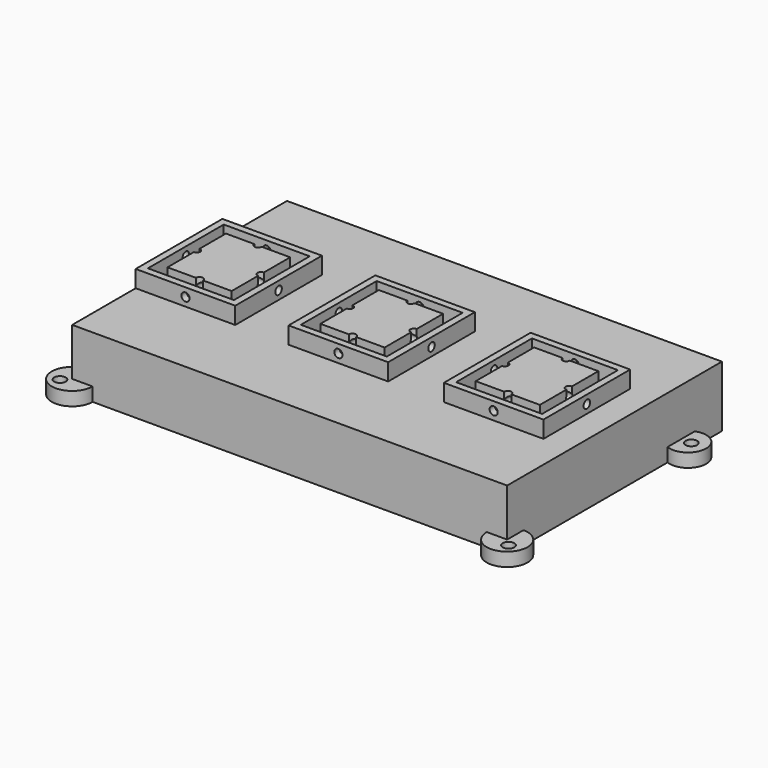
from build123d import *

# Parameters (mm, degrees)
F0_W         = 124
F0_H         = 75
F0_R         = 2
F1_DEPTH     = 2
F2_DEPTH     = 18
F3_W         = 124
F3_H         = 14
F4_DEPTH     = 2
F5_DEPTH     = 5
F6_W         = 124
F6_H         = 1
F7_DEPTH     = 75
F8_W         = 29.3
F8_H         = 31.9
F8_W_2       = 25.3
F8_H_2       = 27.9
F9_DEPTH     = 5
F10_DEPTH    = 4
F11_D        = 3.4
F13_D        = 2.4
F17_D        = 2.4
F17_ON_F15_D = 2.4
F17_ON_F16_D = 2.4
F18_R        = 1.5
F19_DEPTH    = 2


# Not quite as in the source:
# - a feature names something its author has since deleted; it is built from what else it names


with BuildPart() as f1:
    # F0 (on Top) → F1 (new body)
    with BuildSketch(Plane.XY):
        with Locations((1.9529018402, -1.4505029619)):
            Rectangle(F0_W, F0_H)
        with Locations((-53.0470981598, -18.9505029619)):
            Circle(F0_R, mode=Mode.SUBTRACT)
        with Locations((56.9529018402, -18.9505029619)):
            Circle(F0_R, mode=Mode.SUBTRACT)
        with Locations((-53.0470981598, 14.0494970381)):
            Circle(F0_R, mode=Mode.SUBTRACT)
        with Locations((56.9529018402, 14.0494970381)):
            Circle(F0_R, mode=Mode.SUBTRACT)
    extrude(amount=F1_DEPTH)

    # F0 (on Top) → F2 (join)
    with BuildSketch(Plane.XY):
        Polygon((59.9529018402, -40.9505029619), (65.9529018402, -40.9505029619), (65.9529018402, -34.9505029619), (65.9529018402, 18.0494970381), (65.9529018402, 28.0494970381), (65.9529018402, 38.0494970381), (-62.0470981598, 38.0494970381), (-62.0470981598, 28.0494970381), (-62.0470981598, 18.0494970381), (-62.0470981598, -34.9505029619), (-62.0470981598, -40.9505029619), (-56.0470981598, -40.9505029619), align=None)
        with Locations((1.9529018402, -1.4505029619)):
            Rectangle(F0_W, F0_H, mode=Mode.SUBTRACT)
    extrude(amount=F2_DEPTH)

    # F3 (on face) → F4 (cut, through all)
    with BuildSketch(Plane(origin=(0, 38.0494970381, 0), x_dir=(-1, 0, 0), z_dir=(0, 1, 0))):
        with Locations((-1.9529018402, 9)):
            Rectangle(F3_W, F3_H)
    extrude(amount=-F4_DEPTH, mode=Mode.SUBTRACT)

    # F0 (on Top) → F5 (join)
    with BuildSketch(Plane.XY):
        with Locations((-53.0470981598, 14.0494970381)):
            Circle(F0_R)
        with Locations((-53.0470981598, -18.9505029619)):
            Circle(F0_R)
        with Locations((56.9529018402, -18.9505029619)):
            Circle(F0_R)
        with Locations((56.9529018402, 14.0494970381)):
            Circle(F0_R)
    extrude(amount=F5_DEPTH)

    # F6 (on face) → F7 (join, through all)
    with BuildSketch(Plane(origin=(0, -38.9505029619, 0), x_dir=(-1, 0, 0), z_dir=(0, 1, 0))):
        with Locations((-1.9529018402, 17.5)):
            Rectangle(F6_W, F6_H)
    extrude(amount=F7_DEPTH)

    # F8 (on face) → F9 (join)
    with BuildSketch(Plane.XY.offset(18)):
        with Locations((-2.3970981598, -1.6505029619)):
            Rectangle(F8_W, F8_H)
        with Locations((-2.3970981598, -1.6505029619)):
            Rectangle(F8_W_2, F8_H_2, mode=Mode.SUBTRACT)
        with Locations((43.3029018402, -1.6505029619)):
            Rectangle(F8_W, F8_H)
        with Locations((43.3029018402, -1.6505029619)):
            Rectangle(F8_W_2, F8_H_2, mode=Mode.SUBTRACT)
        with Locations((-47.3970981598, -1.6505029619)):
            Rectangle(F8_W, F8_H)
        with Locations((-47.3970981598, -1.6505029619)):
            Rectangle(F8_W_2, F8_H_2, mode=Mode.SUBTRACT)
        with BuildLine():
            Line((7.0529018402, 9.0994970381), (-1.3470981598, 9.0994970381))
            ThreePointArc((-1.3470981598, 9.0994970381), (-2.3970981598, 8.0494970381), (-3.4470981598, 9.0994970381))
            Line((-3.4470981598, 9.0994970381), (-11.8470981598, 9.0994970381))
            Line((-11.8470981598, 9.0994970381), (-11.8470981598, -0.6005029619))
            ThreePointArc((-11.8470981598, -0.6005029619), (-11.1046360395, -0.9080408416), (-10.7970981598, -1.6505029619))
            ThreePointArc((-10.7970981598, -1.6505029619), (-11.1046360395, -2.3929650821), (-11.8470981598, -2.7005029619))
            Line((-11.8470981598, -2.7005029619), (-11.8470981598, -12.4005029619))
            Line((-11.8470981598, -12.4005029619), (-3.4470981598, -12.4005029619))
            ThreePointArc((-3.4470981598, -12.4005029619), (-2.3970981598, -11.3505029619), (-1.3470981598, -12.4005029619))
            Line((-1.3470981598, -12.4005029619), (7.0529018402, -12.4005029619))
            Line((7.0529018402, -12.4005029619), (7.0529018402, -2.7005029619))
            ThreePointArc((7.0529018402, -2.7005029619), (6.0029018402, -1.6505029619), (7.0529018402, -0.6005029619))
            Line((7.0529018402, -0.6005029619), (7.0529018402, 9.0994970381))
        make_face()
        with BuildLine():
            Line((52.7529018402, 9.0994970381), (44.3529018402, 9.0994970381))
            ThreePointArc((44.3529018402, 9.0994970381), (43.3029018402, 8.0494970381), (42.2529018402, 9.0994970381))
            Line((42.2529018402, 9.0994970381), (33.8529018402, 9.0994970381))
            Line((33.8529018402, 9.0994970381), (33.8529018402, -0.6005029619))
            ThreePointArc((33.8529018402, -0.6005029619), (34.5953639605, -0.9080408416), (34.9029018402, -1.6505029619))
            ThreePointArc((34.9029018402, -1.6505029619), (34.5953639605, -2.3929650821), (33.8529018402, -2.7005029619))
            Line((33.8529018402, -2.7005029619), (33.8529018402, -12.4005029619))
            Line((33.8529018402, -12.4005029619), (42.2529018402, -12.4005029619))
            ThreePointArc((42.2529018402, -12.4005029619), (43.3029018402, -11.3505029619), (44.3529018402, -12.4005029619))
            Line((44.3529018402, -12.4005029619), (52.7529018402, -12.4005029619))
            Line((52.7529018402, -12.4005029619), (52.7529018402, -2.7005029619))
            ThreePointArc((52.7529018402, -2.7005029619), (51.7029018402, -1.6505029619), (52.7529018402, -0.6005029619))
            Line((52.7529018402, -0.6005029619), (52.7529018402, 9.0994970381))
        make_face()
        with BuildLine():
            Line((-37.9470981598, 9.0994970381), (-46.3470981598, 9.0994970381))
            ThreePointArc((-46.3470981598, 9.0994970381), (-47.3970981598, 8.0494970381), (-48.4470981598, 9.0994970381))
            Line((-48.4470981598, 9.0994970381), (-56.8470981598, 9.0994970381))
            Line((-56.8470981598, 9.0994970381), (-56.8470981598, -0.6005029619))
            ThreePointArc((-56.8470981598, -0.6005029619), (-56.1046360395, -0.9080408416), (-55.7970981598, -1.6505029619))
            ThreePointArc((-55.7970981598, -1.6505029619), (-56.1046360395, -2.3929650821), (-56.8470981598, -2.7005029619))
            Line((-56.8470981598, -2.7005029619), (-56.8470981598, -12.4005029619))
            Line((-56.8470981598, -12.4005029619), (-48.4470981598, -12.4005029619))
            ThreePointArc((-48.4470981598, -12.4005029619), (-47.3970981598, -11.3505029619), (-46.3470981598, -12.4005029619))
            Line((-46.3470981598, -12.4005029619), (-37.9470981598, -12.4005029619))
            Line((-37.9470981598, -12.4005029619), (-37.9470981598, -2.7005029619))
            ThreePointArc((-37.9470981598, -2.7005029619), (-38.9970981598, -1.6505029619), (-37.9470981598, -0.6005029619))
            Line((-37.9470981598, -0.6005029619), (-37.9470981598, 9.0994970381))
        make_face()
    extrude(amount=F9_DEPTH)

    # F0 (on Top) → F10 (join)
    with BuildSketch(Plane.XY):
        with BuildLine():
            ThreePointArc((-62.0470981598, -34.9505029619), (-66.2897388469, -45.193143649), (-56.0470981598, -40.9505029619))
            Line((-56.0470981598, -40.9505029619), (-62.0470981598, -40.9505029619))
            Line((-62.0470981598, -40.9505029619), (-62.0470981598, -34.9505029619))
        make_face()
        with BuildLine():
            Line((65.9529018402, -34.9505029619), (65.9529018402, -40.9505029619))
            Line((65.9529018402, -40.9505029619), (59.9529018402, -40.9505029619))
            ThreePointArc((59.9529018402, -40.9505029619), (70.1955425273, -45.193143649), (65.9529018402, -34.9505029619))
        make_face()
        with BuildLine():
            Line((65.9529018402, 28.0494970381), (65.9529018402, 18.0494970381))
            ThreePointArc((65.9529018402, 18.0494970381), (73.3380666473, 23.0494970381), (65.9529018402, 28.0494970381))
        make_face()
        with BuildLine():
            ThreePointArc((-62.0470981598, 28.0494970381), (-69.4322629669, 23.0494970381), (-62.0470981598, 18.0494970381))
            Line((-62.0470981598, 18.0494970381), (-62.0470981598, 28.0494970381))
        make_face()
    extrude(amount=F10_DEPTH)

    # F11 (through all)
    with Locations(Plane(origin=(0, 0, 0), x_dir=(1, 0, 0), z_dir=(0, 0, -1))):
        with Locations((-64.0470981598, 42.9505029619), (67.9529018402, 42.9505029619), (68.9529018402, -23.0494970381), (-65.0470981598, -23.0494970381)):
            Hole(F11_D / 2)

    # F13 (through all)
    with Locations(Plane(origin=(-62.0470981598, 0, 0), x_dir=(0, -1, 0), z_dir=(-1, 0, 0))):
        with Locations((1.6505029619, 20.5)):
            Hole(F13_D / 2)

    # F17 (through all)
    with Locations(Plane(origin=(0, 14.2994970381, 0), x_dir=(-1, 0, 0), z_dir=(0, 1, 0))):
        with Locations((-43.3029018402, 20.5)):
            Hole(F17_D / 2)

    # F17 on F15 (through all)
    with Locations(Plane(origin=(0, 14.2994970381, 0), x_dir=(-1, 0, 0), z_dir=(0, 1, 0))):
        with Locations((2.3970981598, 20.5)):
            Hole(F17_ON_F15_D / 2)

    # F17 on F16 (through all)
    with Locations(Plane(origin=(0, 14.2994970381, 0), x_dir=(-1, 0, 0), z_dir=(0, 1, 0))):
        with Locations((47.3970981598, 20.5)):
            Hole(F17_ON_F16_D / 2)

    # F18 (on face) → F19 (cut, through all)
    with BuildSketch(Plane.XY.offset(2)):
        with Locations((46.9529018402, -21.4505029619)):
            Circle(F18_R)
        with Locations((36.9529018402, -21.4505029619)):
            Circle(F18_R)
        with Locations((26.9529018402, -21.4505029619)):
            Circle(F18_R)
        with Locations((16.9529018402, -21.4505029619)):
            Circle(F18_R)
        with Locations((6.9529018402, -21.4505029619)):
            Circle(F18_R)
        with Locations((-3.0470981598, -21.4505029619)):
            Circle(F18_R)
        with Locations((-13.0470981598, -21.4505029619)):
            Circle(F18_R)
        with Locations((-23.0470981598, -21.4505029619)):
            Circle(F18_R)
        with Locations((-33.0470981598, -21.4505029619)):
            Circle(F18_R)
        with Locations((-43.0470981598, -21.4505029619)):
            Circle(F18_R)
        with Locations((-43.0470981598, -11.4505029619)):
            Circle(F18_R)
        with Locations((-33.0470981598, -11.4505029619)):
            Circle(F18_R)
        with Locations((-23.0470981598, -11.4505029619)):
            Circle(F18_R)
        with Locations((-13.0470981598, -11.4505029619)):
            Circle(F18_R)
        with Locations((-3.0470981598, -11.4505029619)):
            Circle(F18_R)
        with Locations((6.9529018402, -11.4505029619)):
            Circle(F18_R)
        with Locations((16.9529018402, -11.4505029619)):
            Circle(F18_R)
        with Locations((26.9529018402, -11.4505029619)):
            Circle(F18_R)
        with Locations((36.9529018402, -11.4505029619)):
            Circle(F18_R)
        with Locations((46.9529018402, -11.4505029619)):
            Circle(F18_R)
        with Locations((46.9529018402, -1.4505029619)):
            Circle(F18_R)
        with Locations((36.9529018402, -1.4505029619)):
            Circle(F18_R)
        with Locations((26.9529018402, -1.4505029619)):
            Circle(F18_R)
        with Locations((16.9529018402, -1.4505029619)):
            Circle(F18_R)
        with Locations((6.9529018402, -1.4505029619)):
            Circle(F18_R)
        with Locations((-3.0470981598, -1.4505029619)):
            Circle(F18_R)
        with Locations((-13.0470981598, -1.4505029619)):
            Circle(F18_R)
        with Locations((-23.0470981598, -1.4505029619)):
            Circle(F18_R)
        with Locations((-33.0470981598, -1.4505029619)):
            Circle(F18_R)
        with Locations((-43.0470981598, -1.4505029619)):
            Circle(F18_R)
        with Locations((-43.0470981598, 8.5494970381)):
            Circle(F18_R)
        with Locations((-33.0470981598, 8.5494970381)):
            Circle(F18_R)
        with Locations((-23.0470981598, 8.5494970381)):
            Circle(F18_R)
        with Locations((-13.0470981598, 8.5494970381)):
            Circle(F18_R)
        with Locations((-3.0470981598, 8.5494970381)):
            Circle(F18_R)
        with Locations((6.9529018402, 8.5494970381)):
            Circle(F18_R)
        with Locations((16.9529018402, 8.5494970381)):
            Circle(F18_R)
        with Locations((26.9529018402, 8.5494970381)):
            Circle(F18_R)
        with Locations((36.9529018402, 8.5494970381)):
            Circle(F18_R)
        with Locations((46.9529018402, 8.5494970381)):
            Circle(F18_R)
        with Locations((46.9529018402, 18.5494970381)):
            Circle(F18_R)
        with Locations((36.9529018402, 18.5494970381)):
            Circle(F18_R)
        with Locations((26.9529018402, 18.5494970381)):
            Circle(F18_R)
        with Locations((16.9529018402, 18.5494970381)):
            Circle(F18_R)
        with Locations((6.9529018402, 18.5494970381)):
            Circle(F18_R)
        with Locations((-3.0470981598, 18.5494970381)):
            Circle(F18_R)
        with Locations((-13.0470981598, 18.5494970381)):
            Circle(F18_R)
        with Locations((-23.0470981598, 18.5494970381)):
            Circle(F18_R)
        with Locations((-33.0470981598, 18.5494970381)):
            Circle(F18_R)
        with Locations((-43.0470981598, 18.5494970381)):
            Circle(F18_R)
    extrude(amount=-F19_DEPTH, mode=Mode.SUBTRACT)


solid = f1.part
